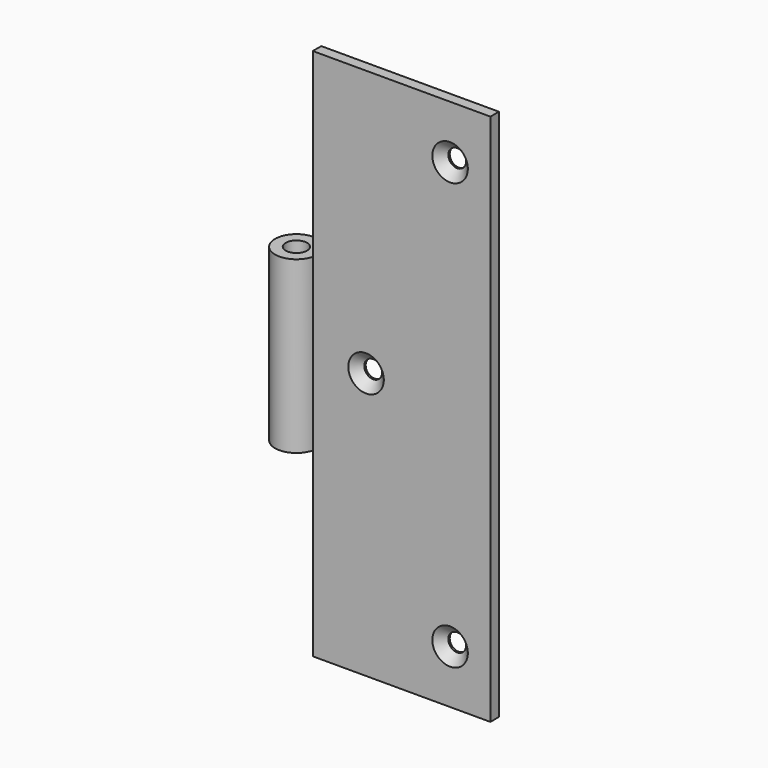
from build123d import *

# Parameters (mm, degrees)
F0_W           = 50
F0_H           = 3
F1_DEPTH       = 150
F3_START       = 51
F2_R           = 6
F2_R_2         = 3
F3_DEPTH       = 48
F5_D           = 5
F5_CSINK_D     = 10
F5_CSINK_ANGLE = 90


# Not quite as in the source:
# - a feature names something its author has since deleted; it is built from what else it names


with BuildPart() as f1:
    # F0 (on Top) → F1 (new body)
    with BuildSketch(Plane.XY):
        with Locations((25, 1.5)):
            Rectangle(F0_W, F0_H)
    extrude(amount=F1_DEPTH)

    # F2 (on Top) → F3 (join)
    with BuildSketch(Plane.XY.offset(F3_START)):
        with Locations((-5.8086630434, 1.5)):
            Circle(F2_R)
        with Locations((-5.8086630434, 1.5)):
            Circle(F2_R_2, mode=Mode.SUBTRACT)
    extrude(amount=F3_DEPTH)

    # F5 (through all)
    with Locations(Plane.XZ):
        with Locations((38.6542826891, 135), (15, 75), (38.6542826891, 15)):
            CounterSinkHole(F5_D / 2, F5_CSINK_D / 2, counter_sink_angle=F5_CSINK_ANGLE)


solid = f1.part
